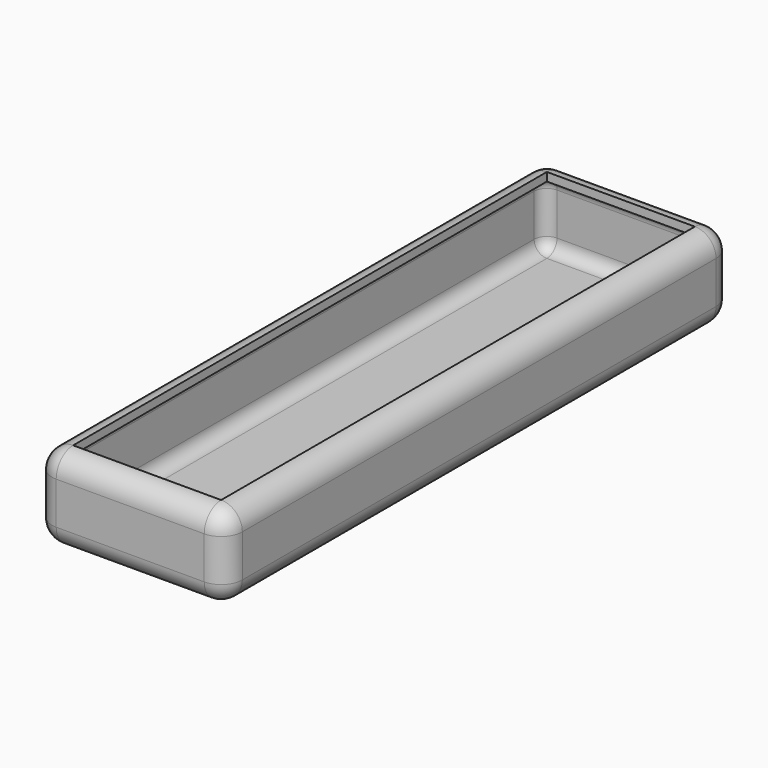
from build123d import *

# Parameters (mm, degrees)
F0_W     = 90
F0_H     = 300
F1_DEPTH = 40
F2_R     = 10
F3_T     = -4


# Not quite as in the source:
# - a shell that OpenCascade refuses in one call is made with other operations: the cavity is built on its own and cut out


with BuildPart() as f1:
    # F0 (on Top) → F1 (new body)
    with BuildSketch(Plane.XY):
        with Locations((-168.3901532187, 84.1299444437)):
            Rectangle(F0_W, F0_H)
    extrude(amount=F1_DEPTH)

    # F2
    f2_edges = [f1.edges().sort_by_distance(p)[0] for p in [
        (-123.390153, 84.129944, 40),
        (-168.390153, -65.870056, 40),
        (-213.390153, 84.129944, 40),
        (-168.390153, 234.129944, 40),
        (-168.390153, -65.870056, 0),
        (-123.390153, 84.129944, 0),
        (-123.390153, 234.129944, 20),
        (-123.390153, -65.870056, 20),
        (-213.390153, -65.870056, 20),
        (-213.390153, 234.129944, 20),
        (-213.390153, 84.129944, 0),
        (-168.390153, 234.129944, 0),
    ]]
    fillet(f2_edges, radius=F2_R)

    # F3: a shell. OpenCascade refuses it in one call, so the cavity is built on its own and cut out:
    # the body offset inwards by the wall thickness, plus a prism from it out through each open face.
    f3_core = offset(f1.part, amount=F3_T, mode=Mode.PRIVATE)
    f3_exits = [f3_core.faces().sort_by_distance(p)[0] for p in [
        (-168.390153, 84.129944, 36),
    ]]
    add(f3_core, mode=Mode.SUBTRACT)
    extrude(f3_exits, amount=-F3_T, mode=Mode.SUBTRACT)


solid = f1.part
